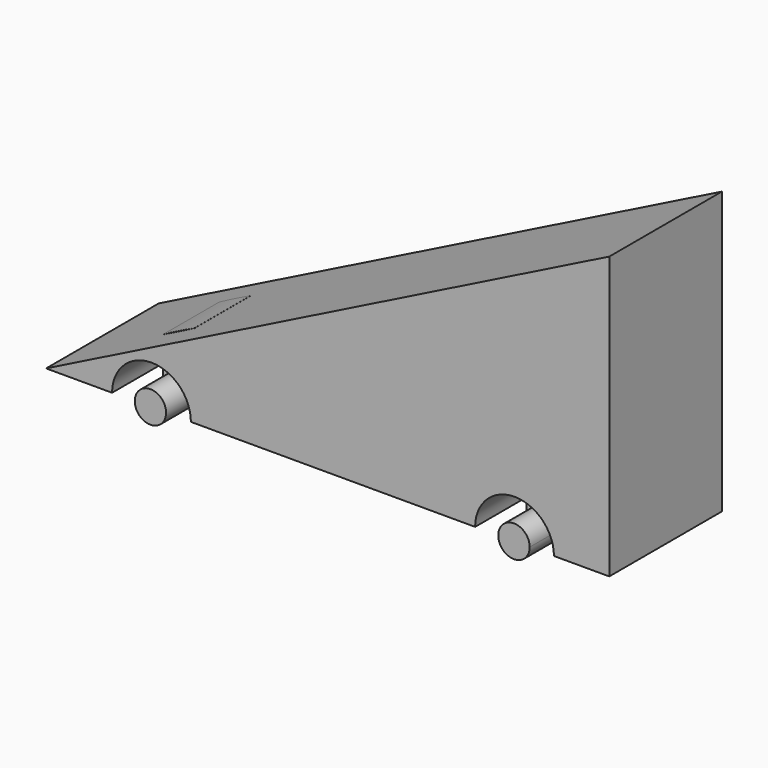
from build123d import *

# Parameters (mm, degrees)
F1_DEPTH    = 6.35
F2_W        = 2.8327330947
F2_H        = 10.4811154306
F3_DEPTH    = 3.175
F4_T4_DEPTH = 134.7141247892
F6_DEPTH    = 6.35


# Not quite as in the source:
# - a fillet or chamfer that OpenCascade refuses, or shapes differently, is made with other operations: its cross-section is extruded or revolved along the edge and cut away or added
# - a feature names something its author has since deleted; it is built from what else it names


with BuildPart() as f1:
    # F0 (on Front) → F1 (new body, symmetric)
    with BuildSketch(Plane.XZ):
        with BuildLine():
            Line((17.3079642735, 0), (17.3079642735, 25.4))
            Line((17.3079642735, 25.4), (-33.4920357265, 0))
            Line((-33.4920357265, 0), (-27.5403555314, 0))
            ThreePointArc((-27.5403555314, 0), (-23.9862389863, 3.5541165451), (-20.4321224411, 0))
            Line((-20.4321224411, 0), (5.2073936615, 0))
            ThreePointArc((5.2073936615, 0), (8.7613936615, 3.554), (12.3153936615, 0))
            Line((12.3153936615, 0), (17.3079642735, 0))
        make_face()
    extrude(amount=F1_DEPTH, both=True)

    # F2 (on Front) → F3 (join, symmetric)
    with BuildSketch(Plane.XZ):
        with Locations((-24.0782387555, 5.2405577153)):
            Rectangle(F2_W, F2_H)
        with Locations((8.7149282917, 5.2405577153)):
            Rectangle(F2_W, F2_H)
    extrude(amount=F3_DEPTH, both=True)

    # F4: fillet of radius 54.0783837972 on 1 edges, made by hand


with BuildPart() as f4_tool2:
    # F4_s3 → F4_t4 (new body)
    with BuildSketch(Plane.XZ.offset(-67.3570623946)):
        with BuildLine():
            ThreePointArc((-25.4946053028, 3.9987152119), (-13.0610727535, 8.8354764656), (0.178219655, 10.4811154306))
            Line((0.178219655, 10.4811154306), (-25.4946053028, 10.4811154306))
            Line((-25.4946053028, 10.4811154306), (-25.4946053028, 3.9987152119))
        make_face()
    extrude(amount=F4_T4_DEPTH)

    split(bisect_by=Plane.YZ.offset(-22.6618722081), keep=Keep.BOTTOM)


with BuildPart() as f1_1:
    add(f1.part)

    # F4_t1: cut F4_tool2
    add(f4_tool2.part, mode=Mode.SUBTRACT)

    # F5 (on Front) → F6 (join, symmetric)
    with BuildSketch(Plane.XZ):
        with BuildLine():
            ThreePointArc((-25.4952833056, 0), (-24.0811295807, -1.4141537249), (-22.6669758558, 0))
            ThreePointArc((-22.6669758558, 0), (-24.0811295807, 1.4141537249), (-25.4952833056, 0))
        make_face()
        with BuildLine():
            ThreePointArc((7.2927195579, 0), (8.7104998529, -1.4270738296), (10.1282801479, 0))
            ThreePointArc((10.1282801479, 0), (8.7104998529, 1.417780295), (7.2927195579, 0))
        make_face()
    extrude(amount=F6_DEPTH, both=True)


solid = f1_1.part
